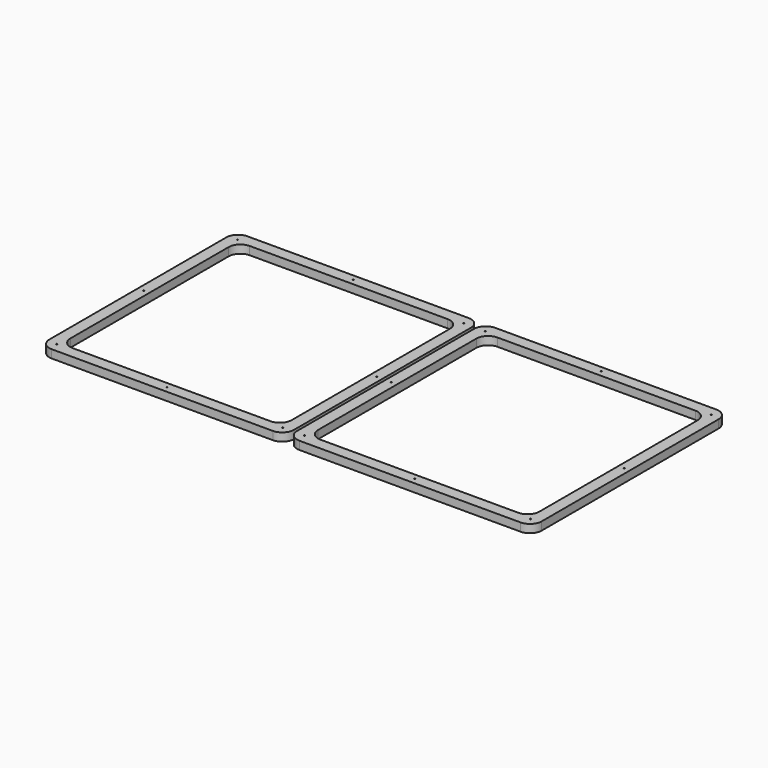
from build123d import *

# Parameters (mm, degrees)
F0_W            = 628
F0_H            = 628
F0_W_2          = 568
F0_H_2          = 568
F1_DEPTH        = 21
F2_R            = 30
F3_R            = 30
F6_R            = 1.5
F7_DEPTH        = 21.001
F7_COPIES_COUNT = 4


# Not quite as in the source:
# - a pattern or mirror of a feature is missing from the dataset's text; its kind, count and spacing are read off the source's solid


with BuildPart() as f1:
    # F0 (on Top) → F1 (new body)
    with BuildSketch(Plane.XY):
        Rectangle(F0_W, F0_H)
        Rectangle(F0_W_2, F0_H_2, mode=Mode.SUBTRACT)
    extrude(amount=F1_DEPTH)

    # F2
    f2_edges = [f1.edges().sort_by_distance(p)[0] for p in [
        (-284, 284, 10.5),
        (284, 284, 10.5),
        (284, -284, 10.5),
        (-284, -284, 10.5),
    ]]
    fillet(f2_edges, radius=F2_R)

    # F3
    f3_edges = [f1.edges().sort_by_distance(p)[0] for p in [
        (-314, -314, 10.5),
        (314, -314, 10.5),
        (314, 314, 10.5),
        (-314, 314, 10.5),
    ]]
    fillet(f3_edges, radius=F3_R)

    # F6 (on face) → F7 (cut, through all)
    with BuildSketch(Plane.XY.offset(21)):
        with Locations((0, 299)):
            Circle(F6_R)
        with Locations((290.2132034356, 290.2132034356)):
            Circle(F6_R)
    f7 = extrude(amount=-F7_DEPTH, mode=Mode.SUBTRACT)

    # F7_copies: F7 ×4 about axis
    f7_copies_axis = Axis((0, 0, 0), (0, 0, 1))
    for i in range(1, F7_COPIES_COUNT):
        add(f7.rotate(f7_copies_axis, i * 360 / F7_COPIES_COUNT), mode=Mode.SUBTRACT)


with BuildPart() as f8_1:
    # F8: instance of F1
    add(f1.part.mirror(Plane(origin=(-318, 0, 10.5), x_dir=(0, -1, 0), z_dir=(-1, 0, 0))))


solid = Compound([f1.part, f8_1.part])
